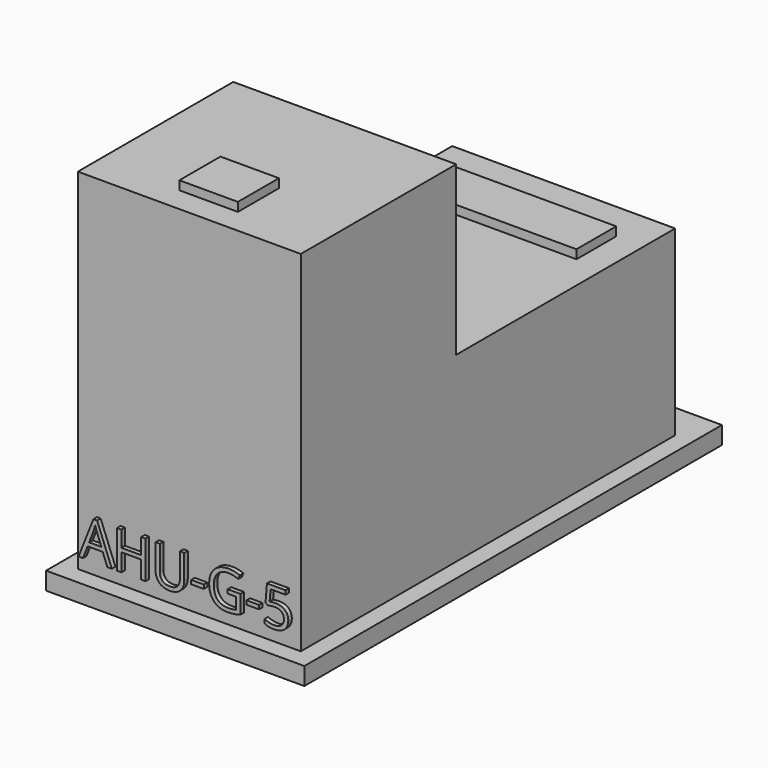
from build123d import *

# Parameters (mm, degrees)
F0_W         = 1282.7
F0_H         = 1047.75
F1_DEPTH     = 2692.4
F2_W         = 1485.9
F2_H         = 101.6
F3_DEPTH     = 101.6
F4_DEPTH     = 2901.95
F5_TEXT_SIZE = 302.8452189432
F6_DEPTH     = 25.4
F7_W         = 965.2
F7_H         = 285.75
F8_DEPTH     = 50.8
F9_W         = 965.2
F9_H         = 285.75
F10_DEPTH    = 50.8
F11_W        = 1282.7
F11_H        = 1117.6
F12_DEPTH    = 965.2
F13_W        = 336.55
F13_H        = 295.275
F14_DEPTH    = 50.8


# Not quite as in the source:
# - Text() gives the source's letters only with a copy of the font that has no kerning and outlines rounded to 1/6400 em; it was checked with that copy


with BuildPart() as f1:
    # F0 (on Front) → F1 (new body)
    with BuildSketch(Plane.XZ):
        with Locations((1.4098696411, -28.5632179465)):
            Rectangle(F0_W, F0_H)
    extrude(amount=F1_DEPTH)

    # F5 (on face) → F6 (join)
    with BuildSketch(Plane.XZ.offset(2692.4)):
        with Locations((-615.5583560467, -470.8269834518)):
            Text('AHU-G-5', F5_TEXT_SIZE, font='Open Sans', text_align=(TextAlign.LEFT, TextAlign.BOTTOM))
    extrude(amount=F6_DEPTH)

    # F7 (on face) → F8 (join)
    with BuildSketch(Plane.XY.offset(495.3117820535)):
        with Locations((1.4098696411, -368.3)):
            Rectangle(F7_W, F7_H)
    extrude(amount=F8_DEPTH)

    # F9 (on face) → F10 (join)
    with BuildSketch(Plane(origin=(0, 0, 0), x_dir=(-1, 0, 0), z_dir=(0, 1, 0))):
        with Locations((-1.4098696411, 50.8117820535)):
            Rectangle(F9_W, F9_H)
    extrude(amount=F10_DEPTH)

    # F11 (on face) → F12 (join)
    with BuildSketch(Plane.XY.offset(495.3117820535)):
        with Locations((1.4098696411, -2133.6)):
            Rectangle(F11_W, F11_H)
    extrude(amount=F12_DEPTH)

    # F13 (on face) → F14 (join)
    with BuildSketch(Plane.XY.offset(1460.5117820535)):
        with Locations((-1.7651303589, -2401.8875)):
            Rectangle(F13_W, F13_H)
    extrude(amount=F14_DEPTH)


with BuildPart() as f3:
    # F2 (on face) → F3 (new body)
    with BuildSketch(Plane.XZ.offset(2692.4)):
        with Locations((1.4098696411, -603.2382179465)):
            Rectangle(F2_W, F2_H)
    extrude(amount=F3_DEPTH)

    # F4 (add): a face of the model
    f4_faces = [f3.faces().sort_by_distance(p)[0] for p in [
        (1.4098696411, -2692.4, -603.2382179465),
    ]]
    extrude(f4_faces, amount=F4_DEPTH)


solid = Compound([f1.part, f3.part])
